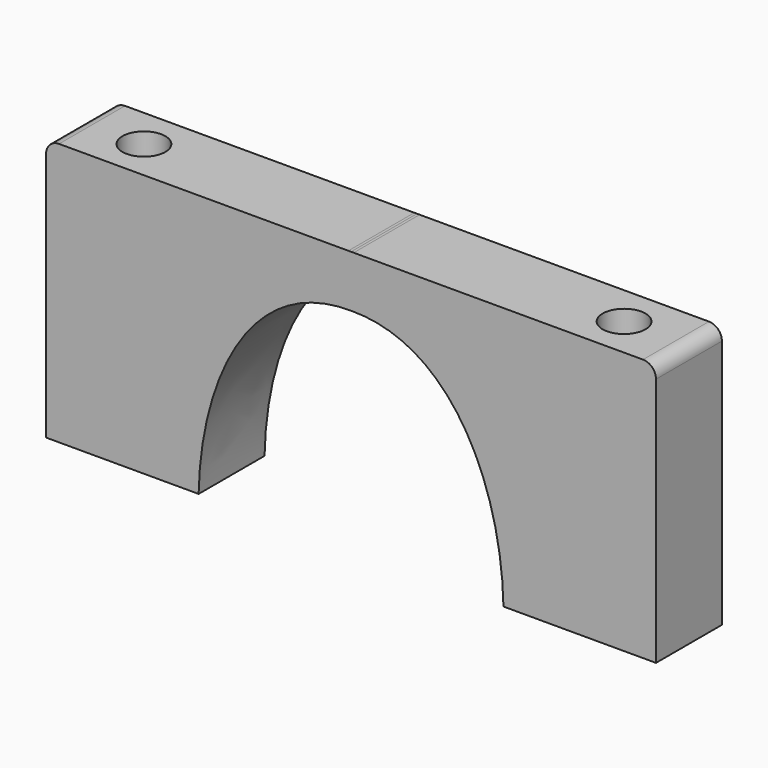
from build123d import *

# Parameters (mm, degrees)
F1_DEPTH = 12.7
F2_R     = 3.302
F3_DEPTH = 41.5002601562
F4_W     = 102.0685225816
F4_H     = 3.4845213629
F5_DEPTH = 25
F6_R     = 2


# Not quite as in the source:
# - ends of sketch curves that miss each other by under 0.0002 mm in the source are joined
# - the dataset's text gives a spline's control points without its knots; the knots are read off the source's solid


with BuildPart() as f1:
    # F0 (on Front) → F1 (new body)
    with BuildSketch(Plane.XZ):
        with BuildLine():
            Line((-8, 0), (0, 0))
            add(Edge.make_bspline(
                [(0, 0), (0, 16.0348825157), (7.430841215, 33.6514413357), (23.5, 33.5)],
                knots=[0, 0, 0, 0, 40.9206549312, 40.9206549312, 40.9206549312, 40.9206549312], degree=3))
            add(Edge.make_bspline(
                [(47, 0), (47, 16.0348825157), (39.569158785, 33.6514413357), (23.5, 33.5)],
                knots=[0, 0, 0, 0, 40.9206549312, 40.9206549312, 40.9206549312, 40.9206549312], degree=3))
            Line((47, 0), (55, 0))
            add(Edge.make_bspline(
                [(55, 0), (55, 2.3133051501), (54.8084752548, 5.6604865088), (54.3346414744, 8.9941225704), (54.1644875118, 10.0000161913)],
                knots=[0, 0, 0, 0, 0.125, 0.1792883855, 0.1792883855, 0.1792883855, 0.1792883855], degree=3))
            add(Edge.make_bspline(
                [(54.1644875118, 10.0000161913), (53.9428588652, 11.3102110198), (53.2041802455, 14.9199242801), (51.403557473, 20.6965522199), (48.312647429, 27.0635606249), (44.7757382973, 31.8590791464), (41.27501086, 35.2044913237), (38.3020149436, 37.39930019), (34.9881581098, 39.2038242784), (31.3670929719, 40.5407901401), (27.6491274865, 41.3170292606), (25.11417344, 41.4919330376), (23.9092731988, 41.5002601562)],
                knots=[0.1792883855, 0.1792883855, 0.1792883855, 0.1792883855, 0.25, 0.375, 0.5, 0.625, 0.6875, 0.75, 0.8125, 0.875, 0.9375, 0.9926226885, 0.9926226885, 0.9926226885, 0.9926226885], degree=3))
            Line((23.9092731988, 41.5002601562), (23.5, 41.5002601562))
            Line((23.5, 41.5002601562), (23.0907268012, 41.5002601562))
            add(Edge.make_bspline(
                [(-7.1644875118, 10.0000161913), (-6.9428588652, 11.3102110198), (-6.2041802455, 14.9199242801), (-4.403557473, 20.6965522199), (-1.312647429, 27.0635606249), (2.2242617027, 31.8590791464), (5.72498914, 35.2044913237), (8.6979850564, 37.39930019), (12.0118418902, 39.2038242784), (15.6329070281, 40.5407901401), (19.3508725135, 41.3170292606), (21.88582656, 41.4919330376), (23.0907268012, 41.5002601562)],
                knots=[0.1792883855, 0.1792883855, 0.1792883855, 0.1792883855, 0.25, 0.375, 0.5, 0.625, 0.6875, 0.75, 0.8125, 0.875, 0.9375, 0.9926226885, 0.9926226885, 0.9926226885, 0.9926226885], degree=3))
            add(Edge.make_bspline(
                [(-8, 0), (-8, 2.3133051501), (-7.8084752548, 5.6604865088), (-7.3346414744, 8.9941225704), (-7.1644875118, 10.0000161913)],
                knots=[0, 0, 0, 0, 0.125, 0.1792883855, 0.1792883855, 0.1792883855, 0.1792883855], degree=3))
        make_face()
        with BuildLine():
            Line((-23.5, 0), (-8, 0))
            add(Edge.make_bspline(
                [(-8, 0), (-8, 2.3133051501), (-7.8084752548, 5.6604865088), (-7.3346414744, 8.9941225704), (-7.1644875118, 10.0000161913)],
                knots=[0, 0, 0, 0, 0.125, 0.1792883855, 0.1792883855, 0.1792883855, 0.1792883855], degree=3))
            Line((-7.1644875118, 10.0000161913), (-23.5, 10))
            Line((-23.5, 10), (-23.5, 0))
        make_face()
        with BuildLine():
            Line((-23.5, 10), (-7.1643917939, 10))
            add(Edge.make_bspline(
                [(-7.1643917939, 10), (-6.9428588652, 11.3102110198), (-6.2041802455, 14.9199242801), (-4.403557473, 20.6965522199), (-1.312647429, 27.0635606249), (2.2242617027, 31.8590791464), (5.72498914, 35.2044913237), (8.6979850564, 37.39930019), (12.0118418902, 39.2038242784), (15.6329070281, 40.5407901401), (19.3508725135, 41.3170292606), (21.88582656, 41.4919330376), (23.0907268012, 41.5002601562)],
                knots=[0.1792883855, 0.1792883855, 0.1792883855, 0.1792883855, 0.25, 0.375, 0.5, 0.625, 0.6875, 0.75, 0.8125, 0.875, 0.9375, 0.9926226885, 0.9926226885, 0.9926226885, 0.9926226885], degree=3))
            Line((23.0907268012, 41.5002601562), (-23.5, 41.5002601562))
            Line((-23.5, 41.5002601562), (-23.5, 10))
        make_face()
        with BuildLine():
            add(Edge.make_bspline(
                [(55, 0), (55, 2.3133051501), (54.8084752548, 5.6604865088), (54.3346414744, 8.9941225704), (54.1644875118, 10.0000161913)],
                knots=[0, 0, 0, 0, 0.125, 0.1792883855, 0.1792883855, 0.1792883855, 0.1792883855], degree=3))
            Line((55, 0), (70.5, 0))
            Line((70.5, 0), (70.5, 10))
            Line((70.5, 10), (54.1644875118, 10.0000161913))
        make_face()
        with BuildLine():
            add(Edge.make_bspline(
                [(23.0907268012, 41.5002601562), (23.2269381476, 41.5012015188), (23.3633657228, 41.5012017791), (23.499999998, 41.5002598872)],
                knots=[0.9926226885, 0.9926226885, 0.9926226885, 0.9926226885, 0.9988541884, 0.9988541884, 0.9988541884, 0.9988541884], degree=3))
            Line((23.0907268012, 41.5002601562), (23.499999998, 41.5002598872))
        make_face()
        with BuildLine():
            add(Edge.make_bspline(
                [(54.1644875118, 10.0000161913), (53.9428588652, 11.3102110198), (53.2041802455, 14.9199242801), (51.403557473, 20.6965522199), (48.312647429, 27.0635606249), (44.7757382973, 31.8590791464), (41.27501086, 35.2044913237), (38.3020149436, 37.39930019), (34.9881581098, 39.2038242784), (31.3670929719, 40.5407901401), (27.6491274865, 41.3170292606), (25.11417344, 41.4919330376), (23.9092731988, 41.5002601562)],
                knots=[0.1792883855, 0.1792883855, 0.1792883855, 0.1792883855, 0.25, 0.375, 0.5, 0.625, 0.6875, 0.75, 0.8125, 0.875, 0.9375, 0.9926226885, 0.9926226885, 0.9926226885, 0.9926226885], degree=3))
            Line((54.1644875118, 10.0000161913), (70.5, 10))
            Line((70.5, 10), (70.5, 41.5002601562))
            Line((70.5, 41.5002601562), (23.9092731988, 41.5002601562))
        make_face()
        with BuildLine():
            add(Edge.make_bspline(
                [(23.9092731988, 41.5002601562), (23.7730618524, 41.5012015188), (23.6366342772, 41.5012017791), (23.500000002, 41.5002598872)],
                knots=[0.9926226885, 0.9926226885, 0.9926226885, 0.9926226885, 0.9988541884, 0.9988541884, 0.9988541884, 0.9988541884], degree=3))
            Line((23.500000002, 41.5002598872), (23.9092731988, 41.5002601562))
        make_face()
    extrude(amount=F1_DEPTH)

    # F2 (on face) → F3 (cut, through all)
    with BuildSketch(Plane.XY.offset(41.5002601562)):
        with Locations((-13.5000000019, -6.35)):
            Circle(F2_R)
        with Locations((60.4999999981, -6.35)):
            Circle(F2_R)
    extrude(amount=-F3_DEPTH, mode=Mode.SUBTRACT)

    # F4 (on Front) → F5 (cut)
    with BuildSketch(Plane.XZ):
        with Locations((22.9078933551, -0.7422606815)):
            Rectangle(F4_W, F4_H)
    extrude(amount=F5_DEPTH, mode=Mode.SUBTRACT)

    # F6
    f6_edges = [f1.edges().sort_by_distance(p)[0] for p in [
        (70.5, -6.35, 41.50026),
        (-23.5, -6.35, 41.50026),
    ]]
    fillet(f6_edges, radius=F6_R)


solid = f1.part
